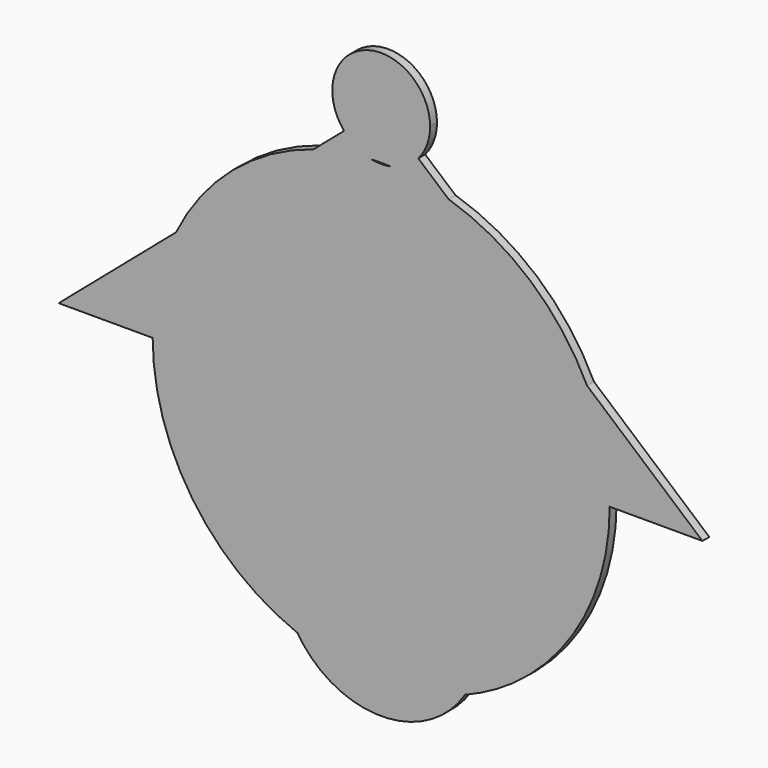
from build123d import *

# Parameters (mm, degrees)
F1_DEPTH = 2


# Not quite as in the source:
# - a feature names something its author has since deleted; it is built from what else it names


with BuildPart() as f1:
    # F0 (on Front) → F1 (new body)
    with BuildSketch(Plane.XZ):
        with BuildLine():
            ThreePointArc((19.4604751144, -49.3491610835), (25.0909627965, -46.7385641336), (30.3780152375, -43.4882280802))
            ThreePointArc((30.3780152375, -43.4882280802), (47.0400422182, -24.5210974354), (53.0476181494, 0))
            Line((53.0476181494, 0), (-53.0476181494, 0))
            ThreePointArc((-53.0476181494, 0), (-43.8541995948, -29.8472606654), (-19.4604751144, -49.3491610835))
            ThreePointArc((-19.4604751144, -49.3491610835), (-6.4361640705, -14.8511496358), (23.054123582, -36.9886383414))
            ThreePointArc((23.054123582, -36.9886383414), (22.1374887057, -43.4248024119), (19.4604751144, -49.3491610835))
        make_face()
        with BuildLine():
            Line((-53.0476181494, 0), (53.0476181494, 0))
            ThreePointArc((53.0476181494, 0), (51.7146557328, 11.817113597), (47.7827569309, 23.0403544115))
            Line((47.7827569309, 23.0403544115), (15.6281781272, 50.6932918615))
            ThreePointArc((15.6281781272, 50.6932918615), (9.002371997, 52.2781702984), (2.2280864718, 53.0008058618))
            ThreePointArc((2.2280864718, 53.0008058618), (0, 52.7800319348), (-2.2280864718, 53.0008058618))
            ThreePointArc((-2.2280864718, 53.0008058618), (-9.0528372764, 52.2694550246), (-15.7260278086, 50.6630224196))
            Line((-15.7260278086, 50.6630224196), (-47.6465335474, 23.3207553961))
            ThreePointArc((-47.6465335474, 23.3207553961), (-51.6797102792, 11.9690156981), (-53.0476181494, 0))
        make_face()
        with BuildLine():
            ThreePointArc((47.7827569309, 23.0403544115), (51.7146557328, 11.817113597), (53.0476181494, 0))
            Line((53.0476181494, 0), (74.573867023, 0))
            Line((74.573867023, 0), (47.7827569309, 23.0403544115))
        make_face()
        with BuildLine():
            ThreePointArc((-19.4604751144, -49.3491610835), (0, -60.0427619235), (19.4604751144, -49.3491610835))
            ThreePointArc((19.4604751144, -49.3491610835), (0, -53.0476181494), (-19.4604751144, -49.3491610835))
        make_face()
        with BuildLine():
            ThreePointArc((-19.4604751144, -49.3491610835), (0, -53.0476181494), (19.4604751144, -49.3491610835))
            ThreePointArc((19.4604751144, -49.3491610835), (22.1374887057, -43.4248024119), (23.054123582, -36.9886383414))
            ThreePointArc((23.054123582, -36.9886383414), (-6.4361640705, -14.8511496358), (-19.4604751144, -49.3491610835))
        make_face()
        with BuildLine():
            Line((15.6281781272, 50.6932918615), (47.7827569309, 23.0403544115))
            ThreePointArc((47.7827569309, 23.0403544115), (34.5891299202, 40.2199189791), (15.6281781272, 50.6932918615))
        make_face()
        with BuildLine():
            Line((-74.8721584678, 0), (-53.0476181494, 0))
            ThreePointArc((-53.0476181494, 0), (-51.6797102792, 11.9690156981), (-47.6465335474, 23.3207553961))
            Line((-47.6465335474, 23.3207553961), (-74.8721584678, 0))
        make_face()
        with BuildLine():
            ThreePointArc((2.2280864718, 53.0008058618), (9.002371997, 52.2781702984), (15.6281781272, 50.6932918615))
            Line((15.6281781272, 50.6932918615), (8.6080503312, 56.7306016959))
            ThreePointArc((8.6080503312, 56.7306016959), (5.730035728, 54.3320712807), (2.2280864718, 53.0008058618))
        make_face()
        with BuildLine():
            ThreePointArc((-15.7260278086, 50.6630224196), (-34.5097127589, 40.2880815704), (-47.6465335474, 23.3207553961))
            Line((-47.6465335474, 23.3207553961), (-15.7260278086, 50.6630224196))
        make_face()
        with BuildLine():
            ThreePointArc((-2.2280864718, 53.0008058618), (0, 53.0476181494), (2.2280864718, 53.0008058618))
            ThreePointArc((2.2280864718, 53.0008058618), (5.730035728, 54.3320712807), (8.6080503312, 56.7306016959))
            Line((8.6080503312, 56.7306016959), (0, 64.1335248947))
            Line((0, 64.1335248947), (-8.6226387996, 56.7475989187))
            ThreePointArc((-8.6226387996, 56.7475989187), (-5.7397015847, 54.3377284437), (-2.2280864718, 53.0008058618))
        make_face()
        with BuildLine():
            Line((0, 64.1335248947), (8.6080503312, 56.7306016959))
            ThreePointArc((8.6080503312, 56.7306016959), (10.6450279761, 60.1857176833), (11.3534929599, 64.1335248947))
            ThreePointArc((11.3534929599, 64.1335248947), (-3.9373045021, 74.7824420063), (-8.6226387996, 56.7475989187))
            Line((-8.6226387996, 56.7475989187), (0, 64.1335248947))
        make_face()
        with BuildLine():
            Line((-8.6226387996, 56.7475989187), (-15.7260278086, 50.6630224196))
            ThreePointArc((-15.7260278086, 50.6630224196), (-9.0528372764, 52.2694550246), (-2.2280864718, 53.0008058618))
            ThreePointArc((-2.2280864718, 53.0008058618), (-5.7397015847, 54.3377284437), (-8.6226387996, 56.7475989187))
        make_face()
    extrude(amount=F1_DEPTH)


solid = f1.part
